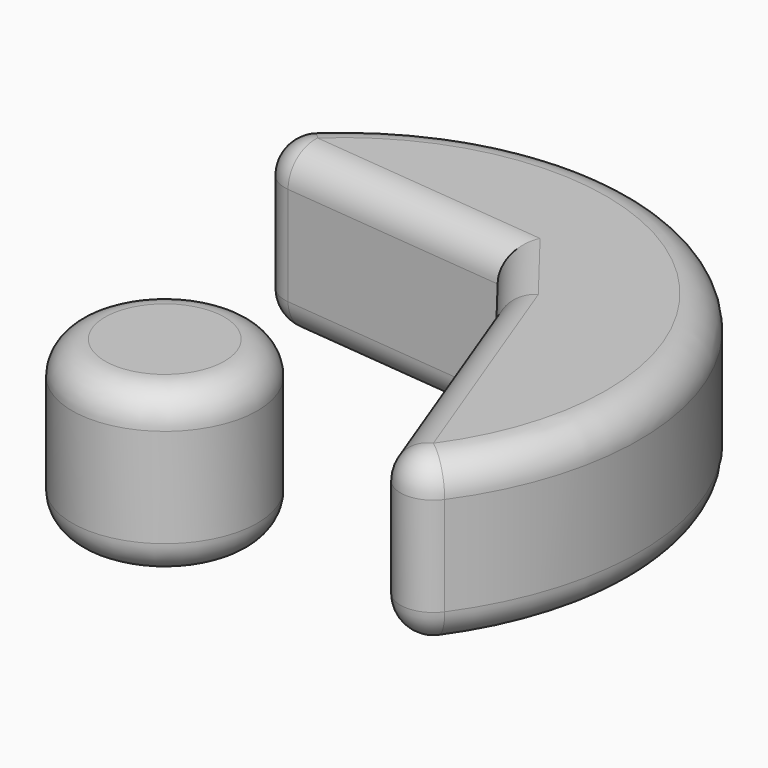
from build123d import *

# Parameters (mm, degrees)
F1_DEPTH = 25.4
F0_R     = 14.2835162245
F3_R     = 5.08
F4_R     = 5.08


# Not quite as in the source:
# - a feature of the source that left no trace in its solid (it failed there, or was rolled back) is left out


with BuildPart() as f1:
    # F0 (on Top) → F1 (new body)
    with BuildSketch(Plane.XY):
        with BuildLine():
            ThreePointArc((40.4053583261, -10.6703329711), (38.948965984, 57.412745276), (-28.5416923943, 48.3332269014))
            Line((-28.5416923943, 48.3332269014), (16.2010799613, 43.8748665274))
            Line((16.2010799613, 43.8748665274), (23.3559507397, 34.6526309968))
            Line((23.3559507397, 34.6526309968), (40.4053583261, -10.6703329711))
        make_face()
    extrude(amount=F1_DEPTH)

    # F4
    f4_edges = [f1.edges().sort_by_distance(p)[0] for p in [
        (38.948966, 57.412745, 0),
        (19.778515, 39.263749, 0),
        (31.880655, 11.991149, 0),
        (-6.170306, 46.104047, 0),
        (19.778515, 39.263749, 25.4),
        (40.405358, -10.670333, 12.7),
        (31.880655, 11.991149, 25.4),
        (-28.541692, 48.333227, 12.7),
        (38.948966, 57.412745, 25.4),
        (-6.170306, 46.104047, 25.4),
    ]]
    fillet(f4_edges, radius=F4_R)


with BuildPart() as f1b:
    # F0 (on Top) → F1, piece 2 (new body)
    with BuildSketch(Plane.XY):
        Circle(F0_R)
    extrude(amount=F1_DEPTH)

    # F3
    f3_edges = [f1b.edges().sort_by_distance(p)[0] for p in [
        (-14.283516, 0, 0),
        (-14.283516, 0, 25.4),
        (14.283516, 0, 12.7),
    ]]
    fillet(f3_edges, radius=F3_R)


solid = Compound([f1.part, f1b.part])
